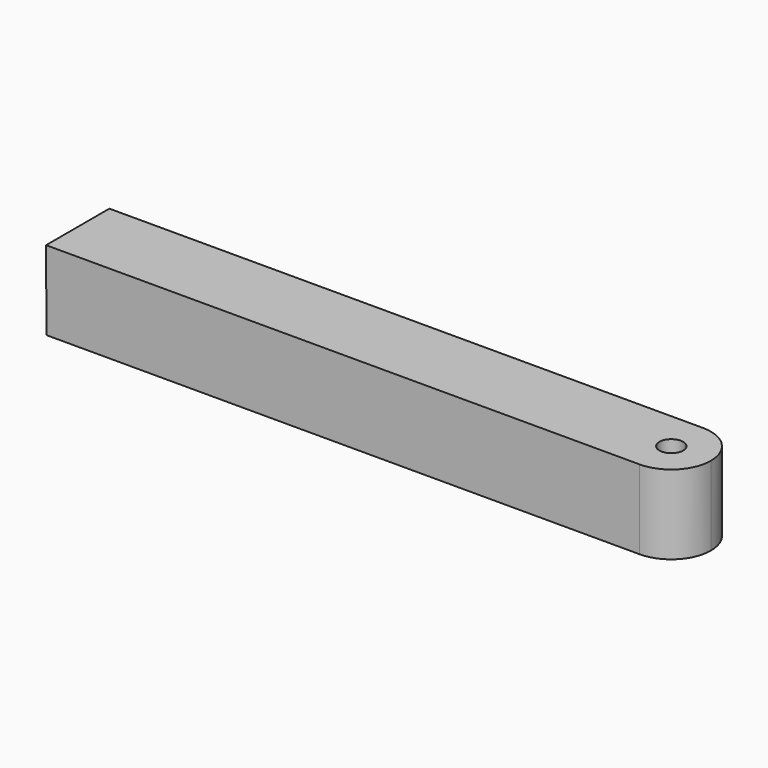
from build123d import *

# Parameters (mm, degrees)
F1_DEPTH = 10
F3_D     = 3
F4_R     = 4.99999


# Not quite as in the source:
# - a fillet or chamfer is up to 0.001 mm smaller than in the source, because OpenCascade refuses the exact size


with BuildPart() as f1:
    # F0 (on Front) → F1 (new body)
    with BuildSketch(Plane.XZ):
        Polygon((-25.8799286838, 0), (44.1200713162, 0), (44.1200713162, 10), (-25.9238125384, 10), (-35.9238125384, 10), (-35.8799286838, 0), align=None)
    extrude(amount=F1_DEPTH)

    # F3 (through all)
    with Locations(Plane.XY.offset(10)):
        with Locations((39.1200713162, -5)):
            Hole(F3_D / 2)

    # F4 (radius 5 in the source; OpenCascade refuses exactly that, so slightly less here)
    f4_edges = [f1.edges().sort_by_distance(p)[0] for p in [
        (44.120071, -10, 5),
        (44.120071, 0, 5),
    ]]
    fillet(f4_edges, radius=F4_R)


solid = f1.part
